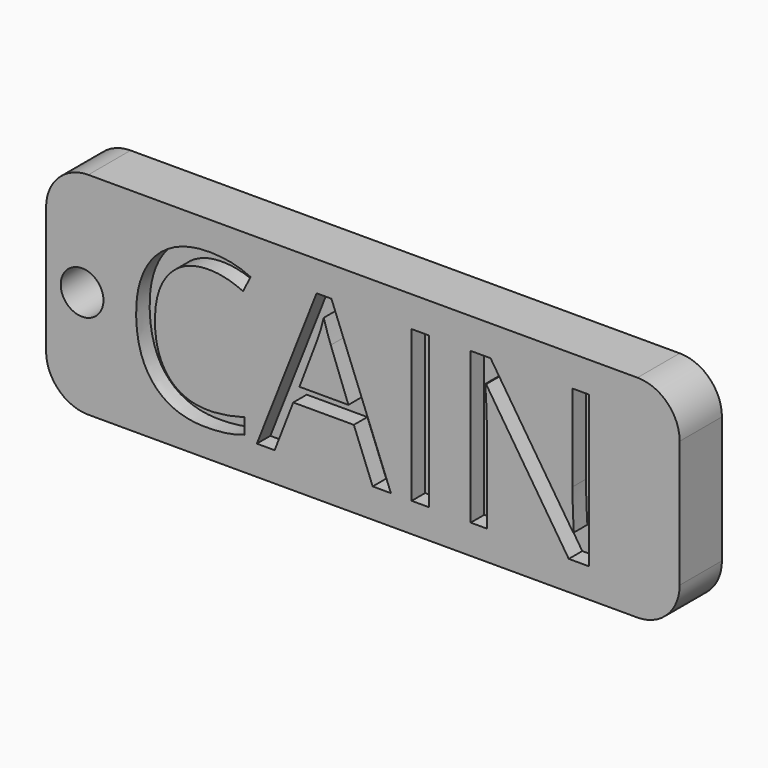
from build123d import *

# Parameters (mm, degrees)
F0_W         = 76.2
F0_H         = 25.4
F1_DEPTH     = 6.35
F2_R         = 5.08
F3_TEXT_SIZE = 25.47393346
F4_DEPTH     = 2.032
F5_R         = 2.568164757
F6_DEPTH     = 25.4


# Not quite as in the source:
# - Text() gives the source's letters only with a copy of the font that has no kerning and outlines rounded to 1/6400 em; it was checked with that copy


with BuildPart() as f1:
    # F0 (on Front) → F1 (new body)
    with BuildSketch(Plane.XZ):
        Rectangle(F0_W, F0_H)
    extrude(amount=-F1_DEPTH)

    # F2
    f2_edges = [f1.edges().sort_by_distance(p)[0] for p in [
        (-38.1, 3.175, 12.7),
        (-38.1, 3.175, -12.7),
        (38.1, 3.175, 12.7),
        (38.1, 3.175, -12.7),
    ]]
    fillet(f2_edges, radius=F2_R)

    # F3 (on Front) → F4 (cut)
    with BuildSketch(Plane.XZ):
        with Locations((-28.8253478308, -9.1706160456)):
            Text('CAIN', F3_TEXT_SIZE, font='Open Sans', text_align=(TextAlign.LEFT, TextAlign.BOTTOM))
    extrude(amount=-F4_DEPTH, mode=Mode.SUBTRACT)

    # F5 (on Front) → F6 (cut)
    with BuildSketch(Plane.XZ):
        with Locations((-33.769518137, 0)):
            Circle(F5_R)
    extrude(amount=-F6_DEPTH, mode=Mode.SUBTRACT)


solid = f1.part
